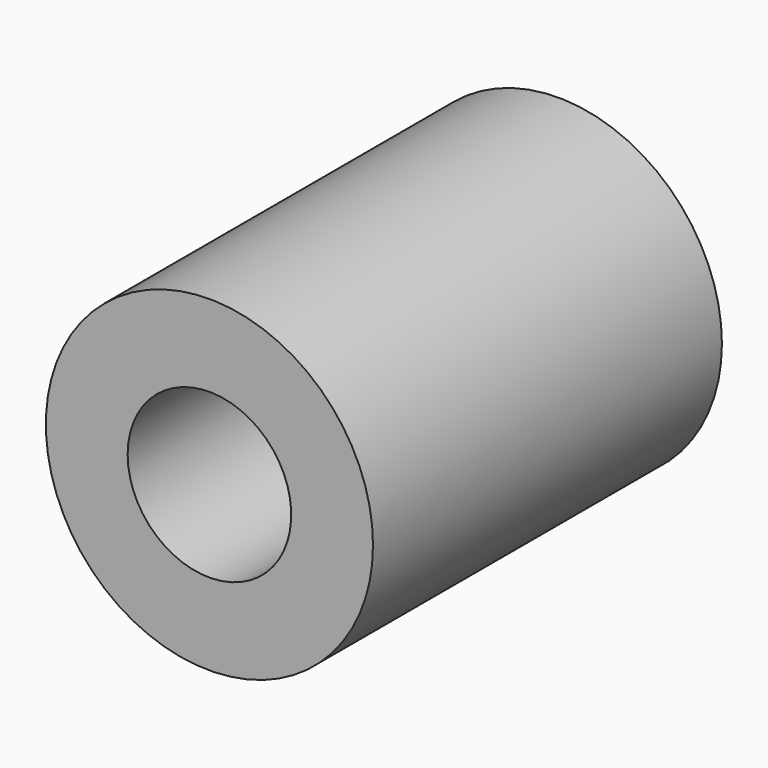
from build123d import *

# Parameters (mm, degrees)
F0_R     = 9.525
F1_DEPTH = 25.4
F3_D     = 9.525


# Not quite as in the source:
# - the program builds the solid bodies; features that only make, move or delete a surface that nothing else refers to are left out


with BuildPart() as f1:
    # F0 (on Front) → F1 (new body)
    with BuildSketch(Plane.XZ):
        Circle(F0_R)
    extrude(amount=F1_DEPTH)

    # F3 (through all)
    with Locations(Plane(origin=(0, 0, 0), x_dir=(1, 0, 0), z_dir=(0, 1, 0))):
        with Locations((0, 0)):
            Hole(F3_D / 2)


solid = f1.part
